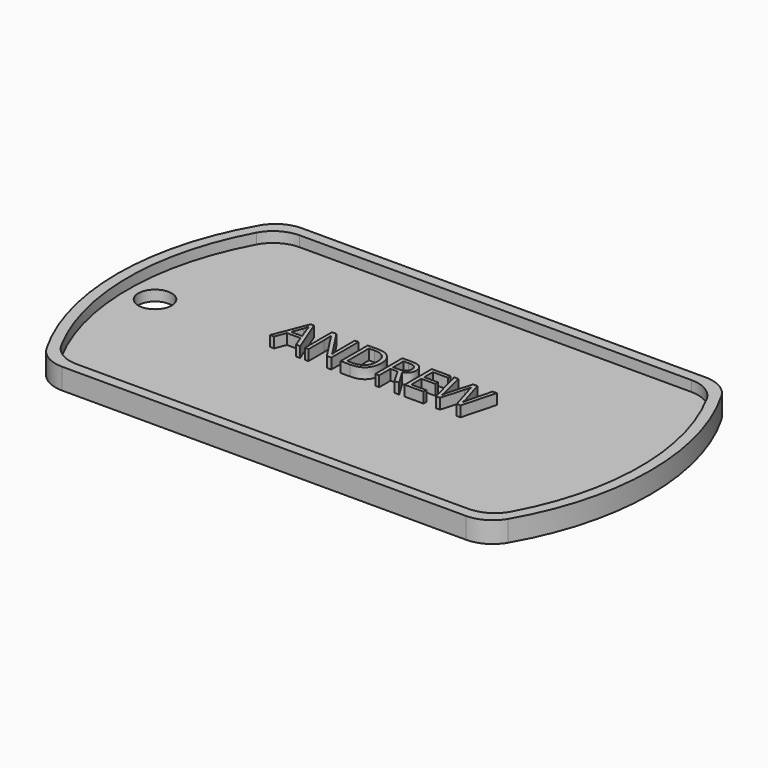
from build123d import *

# Parameters (mm, degrees)
F1_DEPTH     = 1
F3_DEPTH     = 1
F4_R         = 1.5875
F5_DEPTH     = 1
F6_TEXT_SIZE = 4.5258513031
F7_DEPTH     = 1


# Not quite as in the source:
# - Text() gives the source's letters only with a copy of the font that has no kerning and outlines rounded to 1/6400 em; it was checked with that copy


with BuildPart() as f1:
    # F0 (on Top) → F1 (new body)
    with BuildSketch(Plane.XY):
        with BuildLine():
            ThreePointArc((-19.2474145991, 14.2875), (-20.8349145991, 13.862130657), (-21.9970452561, 12.7))
            ThreePointArc((-21.9970452561, 12.7), (-25.4, 0), (-21.9970452561, -12.7))
            ThreePointArc((-21.9970452561, -12.7), (-20.8349145991, -13.862130657), (-19.2474145991, -14.2875))
            Line((-19.2474145991, -14.2875), (19.2474145991, -14.2875))
            ThreePointArc((19.2474145991, -14.2875), (20.8349145991, -13.862130657), (21.9970452561, -12.7))
            ThreePointArc((21.9970452561, -12.7), (25.4, 0), (21.9970452561, 12.7))
            ThreePointArc((21.9970452561, 12.7), (20.8349145991, 13.862130657), (19.2474145991, 14.2875))
            Line((19.2474145991, 14.2875), (-19.2474145991, 14.2875))
        make_face()
    extrude(amount=F1_DEPTH)

    # F2 (on face) → F3 (join)
    with BuildSketch(Plane.XY.offset(1)):
        with BuildLine():
            Line((19.2474145991, 14.2875), (-19.2474145991, 14.2875))
            ThreePointArc((-19.2474145991, 14.2875), (-20.8349145991, 13.862130657), (-21.9970452561, 12.7))
            ThreePointArc((-21.9970452561, 12.7), (-25.4, 0), (-21.9970452561, -12.7))
            ThreePointArc((-21.9970452561, -12.7), (-20.8349145991, -13.862130657), (-19.2474145991, -14.2875))
            Line((-19.2474145991, -14.2875), (19.2474145991, -14.2875))
            ThreePointArc((19.2474145991, -14.2875), (20.8349145991, -13.862130657), (21.9970452561, -12.7))
            ThreePointArc((21.9970452561, -12.7), (25.4, 0), (21.9970452561, 12.7))
            ThreePointArc((21.9970452561, 12.7), (20.8349145991, 13.862130657), (19.2474145991, 14.2875))
        make_face()
        with BuildLine():
            ThreePointArc((-21.4526124879, 11.6252061249), (-20.2856017842, 12.8404540819), (-18.6611352482, 13.2875))
            Line((-18.6611352482, 13.2875), (18.6611352482, 13.2875))
            ThreePointArc((18.6611352482, 13.2875), (20.2856017842, 12.8404540819), (21.4526124879, 11.6252061249))
            ThreePointArc((21.4526124879, 11.6252061249), (24.4, 0), (21.4526124879, -11.6252061249))
            ThreePointArc((21.4526124879, -11.6252061249), (20.2856017842, -12.8404540819), (18.6611352482, -13.2875))
            Line((18.6611352482, -13.2875), (-18.6611352482, -13.2875))
            ThreePointArc((-18.6611352482, -13.2875), (-20.2856017842, -12.8404540819), (-21.4526124879, -11.6252061249))
            ThreePointArc((-21.4526124879, -11.6252061249), (-24.4, 0), (-21.4526124879, 11.6252061249))
        make_face(mode=Mode.SUBTRACT)
    extrude(amount=F3_DEPTH)

    # F4 (on face) → F5 (cut)
    with BuildSketch(Plane.XY.offset(1)):
        with Locations((-21.821282804, 0)):
            Circle(F4_R)
    extrude(amount=-F5_DEPTH, mode=Mode.SUBTRACT)

    # F6 (on face) → F7 (join)
    with BuildSketch(Plane.XY.offset(1)):
        with Locations((-10.3466827422, -0.6305378629)):
            Text('ANDREW', F6_TEXT_SIZE, font='Open Sans', text_align=(TextAlign.LEFT, TextAlign.BOTTOM))
    extrude(amount=F7_DEPTH)


solid = f1.part
